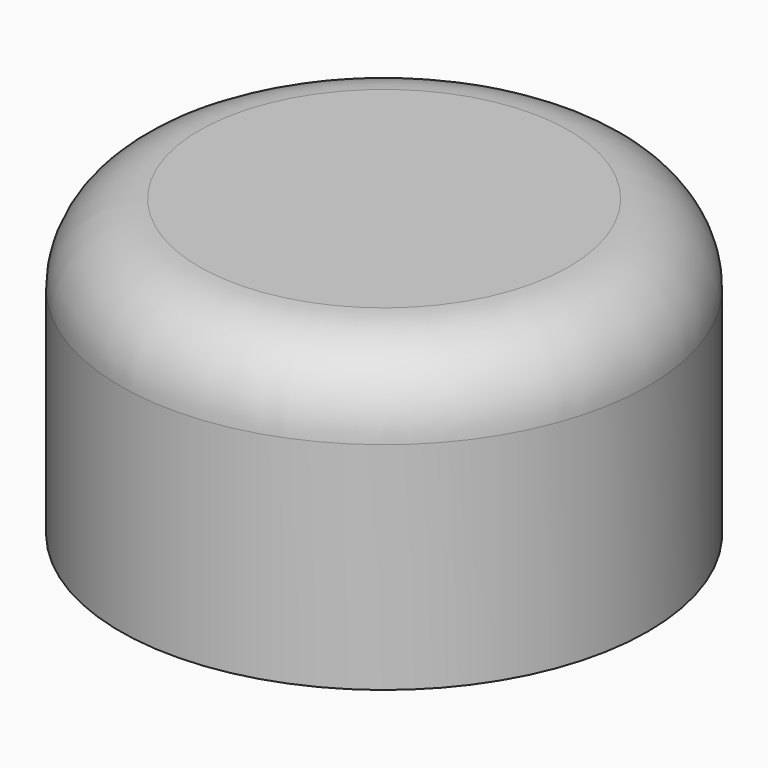
from build123d import *

# Parameters (mm, degrees)
F0_R     = 25.4
F0_R_2   = 23.7717418162
F1_DEPTH = 25.4
F2_R     = 25.4
F2_R_2   = 23.7717418162
F3_DEPTH = 3
F4_R     = 7.62


# Not quite as in the source:
# - a fillet or chamfer that OpenCascade refuses, or shapes differently, is made with other operations: its cross-section is extruded or revolved along the edge and cut away or added


with BuildPart() as f1:
    # F0 (on Top) → F1 (new body)
    with BuildSketch(Plane.XY):
        Circle(F0_R)
        Circle(F0_R_2, mode=Mode.SUBTRACT)
    extrude(amount=F1_DEPTH)

    # F2 (on face) → F3 (join)
    with BuildSketch(Plane.XY.offset(25.4)):
        Circle(F2_R)
        Circle(F2_R_2, mode=Mode.SUBTRACT)
        Circle(F2_R)
    extrude(amount=F3_DEPTH)

    # F4
    f4_edges = [f1.edges().sort_by_distance(p)[0] for p in [
        (-25.4, 0, 28.4),
    ]]
    fillet(f4_edges, radius=F4_R)

    # F5: fillet of radius 5.08 on 1 edges, made by hand

    # F5_s1 → F5_t2 (revolve, cut)
    with BuildSketch(Plane.XZ):
        with BuildLine():
            ThreePointArc((25.4, 0), (24.1965700457, 1.6935203443), (23.7717418162, 3.7271810305))
            Line((23.7717418162, 3.7271810305), (23.7717418162, 0))
            Line((23.7717418162, 0), (25.4, 0))
        make_face()
    revolve(axis=Axis((0, 0, 0), (0, 0, 1)), mode=Mode.SUBTRACT)


solid = f1.part
